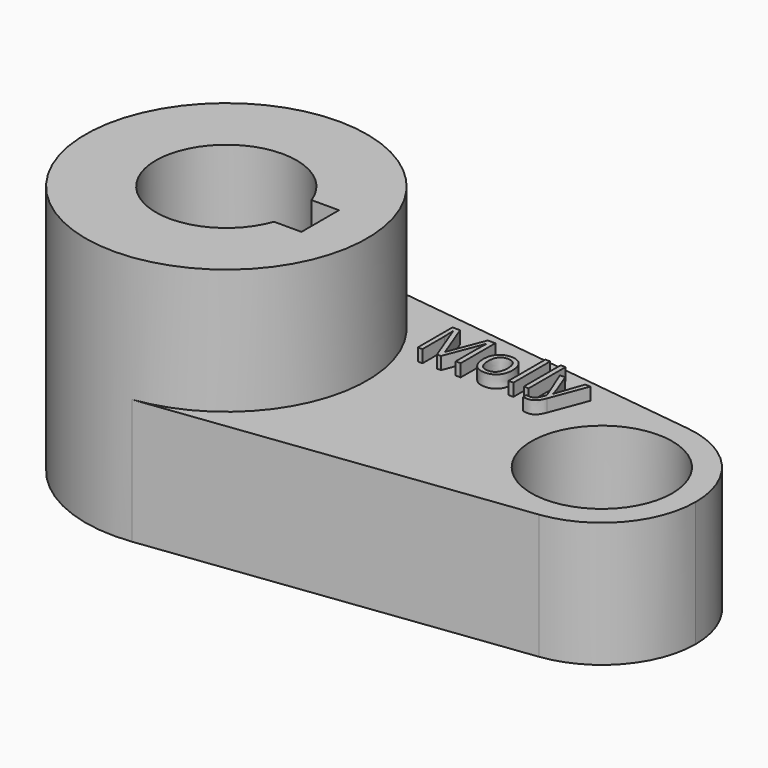
from build123d import *

# Parameters (mm, degrees)
F0_R         = 14.2875
F1_DEPTH     = 25.4
F2_DEPTH     = 50.8
F3_TEXT_SIZE = 12.3032211189
F4_DEPTH     = 2.54


# Not quite as in the source:
# - Text() gives the source's letters only with a copy of the font that has no kerning and outlines rounded to 1/6400 em; it was checked with that copy


with BuildPart() as f1:
    # F0 (on Top) → F1 (new body)
    with BuildSketch(Plane.XY):
        with BuildLine():
            ThreePointArc((3.571875, -28.3508788926), (21.43125, -18.9005859284), (28.575, 0))
            ThreePointArc((28.575, 0), (21.43125, 18.9005859284), (3.571875, 28.3508788926))
            ThreePointArc((3.571875, 28.3508788926), (-28.575, 0), (3.571875, -28.3508788926))
        make_face()
        with BuildLine():
            ThreePointArc((-13.4703841816, 4.7625), (0, 14.2875), (13.4703841816, 4.7625))
            Line((13.4703841816, 4.7625), (19.05, 4.7625))
            Line((19.05, 4.7625), (19.05, -4.7625))
            Line((19.05, -4.7625), (13.4703841816, -4.7625))
            ThreePointArc((13.4703841816, -4.7625), (0, -14.2875), (-13.4703841816, -4.7625))
            Line((-13.4703841816, -4.7625), (-19.05, -4.7625))
            Line((-19.05, -4.7625), (-19.05, 4.7625))
            Line((-19.05, 4.7625), (-13.4703841816, 4.7625))
        make_face(mode=Mode.SUBTRACT)
        with BuildLine():
            ThreePointArc((-13.4703841816, -4.7625), (-14.2875, 0), (-13.4703841816, 4.7625))
            Line((-13.4703841816, 4.7625), (-19.05, 4.7625))
            Line((-19.05, 4.7625), (-19.05, -4.7625))
            Line((-19.05, -4.7625), (-13.4703841816, -4.7625))
        make_face()
        with BuildLine():
            ThreePointArc((3.571875, 28.3508788926), (21.43125, 18.9005859284), (28.575, 0))
            ThreePointArc((28.575, 0), (21.43125, -18.9005859284), (3.571875, -28.3508788926))
            Line((3.571875, -28.3508788926), (78.58125, -18.9005859284))
            ThreePointArc((78.58125, -18.9005859284), (57.15, 0), (78.58125, 18.9005859284))
            Line((78.58125, 18.9005859284), (3.571875, 28.3508788926))
        make_face()
        with BuildLine():
            ThreePointArc((95.25, 0), (90.4875, 12.6003906189), (78.58125, 18.9005859284))
            ThreePointArc((78.58125, 18.9005859284), (57.15, 0), (78.58125, -18.9005859284))
            ThreePointArc((78.58125, -18.9005859284), (90.4875, -12.6003906189), (95.25, 0))
        make_face()
        with Locations((76.2, 0)):
            Circle(F0_R, mode=Mode.SUBTRACT)
    extrude(amount=F1_DEPTH)

    # F0 (on Top) → F2 (join)
    with BuildSketch(Plane.XY):
        with BuildLine():
            ThreePointArc((3.571875, -28.3508788926), (21.43125, -18.9005859284), (28.575, 0))
            ThreePointArc((28.575, 0), (21.43125, 18.9005859284), (3.571875, 28.3508788926))
            ThreePointArc((3.571875, 28.3508788926), (-28.575, 0), (3.571875, -28.3508788926))
        make_face()
        with BuildLine():
            ThreePointArc((-13.4703841816, 4.7625), (0, 14.2875), (13.4703841816, 4.7625))
            Line((13.4703841816, 4.7625), (19.05, 4.7625))
            Line((19.05, 4.7625), (19.05, -4.7625))
            Line((19.05, -4.7625), (13.4703841816, -4.7625))
            ThreePointArc((13.4703841816, -4.7625), (0, -14.2875), (-13.4703841816, -4.7625))
            Line((-13.4703841816, -4.7625), (-19.05, -4.7625))
            Line((-19.05, -4.7625), (-19.05, 4.7625))
            Line((-19.05, 4.7625), (-13.4703841816, 4.7625))
        make_face(mode=Mode.SUBTRACT)
        with BuildLine():
            ThreePointArc((-13.4703841816, -4.7625), (-14.2875, 0), (-13.4703841816, 4.7625))
            Line((-13.4703841816, 4.7625), (-19.05, 4.7625))
            Line((-19.05, 4.7625), (-19.05, -4.7625))
            Line((-19.05, -4.7625), (-13.4703841816, -4.7625))
        make_face()
    extrude(amount=F2_DEPTH)

    # F3 (on face) → F4 (join)
    with BuildSketch(Plane.XY.offset(25.4)):
        with Locations((29.5715820201, 10.1049677136)):
            Text('Molly', F3_TEXT_SIZE, font='Open Sans', text_align=(TextAlign.LEFT, TextAlign.BOTTOM))
    extrude(amount=F4_DEPTH)


solid = f1.part
